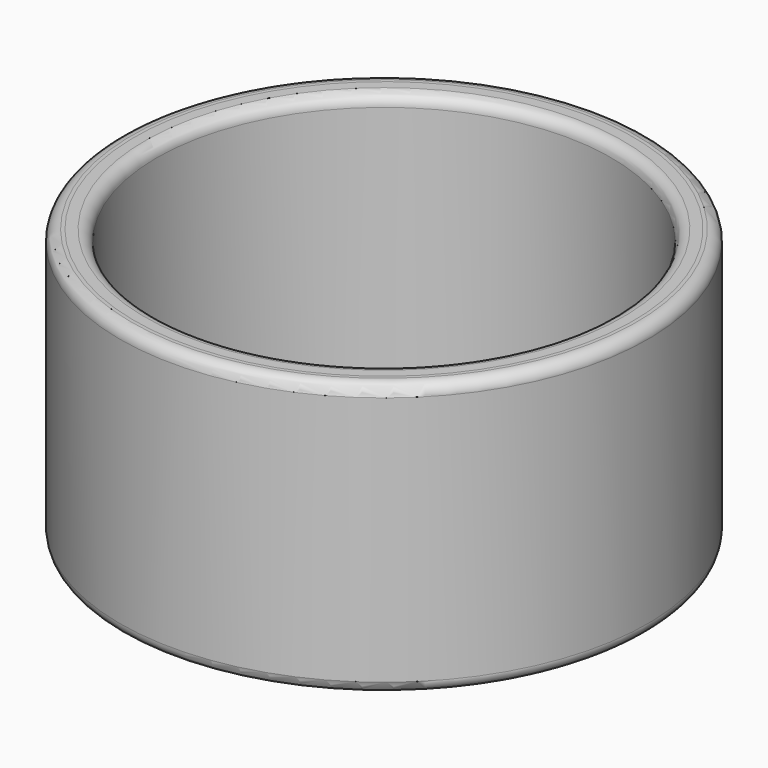
from build123d import *

# Parameters (mm, degrees)
F2_W          = 0.3
F2_H          = 10
F5_ANGLE_BACK = 48.7028489575
F5_ANGLE      = 97.405697915
F6_ANGLE_BACK = 2
F6_ANGLE      = 4
F7_R          = 0.5
F7_2_R        = 0.5


with BuildPart() as f3:
    # F2 (on Right) → F3 (revolve)
    with BuildSketch(Plane.YZ):
        Polygon((10.95, 12), (10.95, 11), (10.95, 1), (10.65, 1), (10, 1), (10, 0), (11.6, 0), (11.6, 2.7), (11.6, 9.3), (11.6, 12), align=None)
    revolve(axis=Axis((0, 0, 13.9442766085), (0, 0, -1)))

    # F2 (on Right) → F6 (revolve)
    with BuildSketch(Plane.YZ, mode=Mode.PRIVATE) as f6_sk:
        Polygon((11.9, 9), (11.6, 9.3), (11.6, 2.7), (11.9, 3), align=None)
    revolve(f6_sk.sketch.rotate(Axis((0, 0, 13.9442766085), (0, 0, -1)), -F6_ANGLE_BACK), axis=Axis((0, 0, 13.9442766085), (0, 0, -1)), revolution_arc=F6_ANGLE)

    # F7
    f7_edges = [f3.edges().sort_by_distance(p)[0] for p in [
        (0, -11.6, 12),
        (0, -10, 0),
        (0, -11.6, 0),
    ]]
    fillet(f7_edges, radius=F7_R)


with BuildPart() as f4:
    # F2 (on Right) → F4 (revolve)
    with BuildSketch(Plane.YZ):
        Polygon((10.65, 1), (10.65, 11), (10.95, 11), (10.95, 12), (10, 12), (10, 1), align=None)
        with Locations((10.8, 6)):
            Rectangle(F2_W, F2_H)
    revolve(axis=Axis((0, 0, 13.9442766085), (0, 0, -1)))

    # F2 (on Right) → F5 (revolve, cut)
    with BuildSketch(Plane.YZ, mode=Mode.PRIVATE) as f5_sk:
        with Locations((10.8, 6)):
            Rectangle(F2_W, F2_H)
        with Locations((-10.8, 6)):
            Rectangle(F2_W, F2_H)
    revolve(f5_sk.sketch.rotate(Axis((0, 0, 13.9442766085), (0, 0, -1)), -F5_ANGLE_BACK), axis=Axis((0, 0, 13.9442766085), (0, 0, -1)), revolution_arc=F5_ANGLE, mode=Mode.SUBTRACT)

    # F7#2
    f7_2_edges = [f4.edges().sort_by_distance(p)[0] for p in [
        (0, -10, 12),
    ]]
    fillet(f7_2_edges, radius=F7_2_R)


solid = Compound([f3.part, f4.part])
